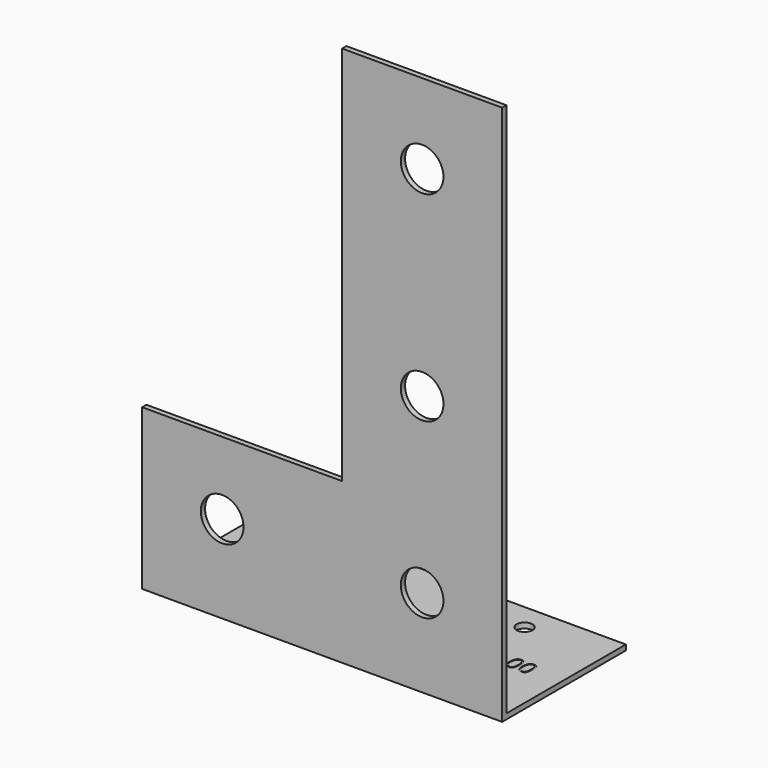
from build123d import *

# Parameters (mm, degrees)
F0_R         = 4
F0_W         = 67.5
F0_H         = 1
F1_DEPTH     = 1
F2_DEPTH     = 28
F3_R         = 1.5
F4_DEPTH     = 1
F5_TEXT_SIZE = 4.1666666667
F6_DEPTH     = 0.1


# Not quite as in the source:
# - Text() gives the source's letters only with a copy of the font that has no kerning and outlines rounded to 1/6400 em; it was checked with that copy


with BuildPart() as f1:
    # F0 (on Front) → F1 (new body)
    with BuildSketch(Plane.XZ):
        Polygon((0, 0), (-37.5, 0), (-37.5, -29), (30, -29), (30, 71.4), (0, 71.4), align=None)
        with Locations((-22.5, -13.6)):
            Circle(F0_R, mode=Mode.SUBTRACT)
        with Locations((15, -13.6)):
            Circle(F0_R, mode=Mode.SUBTRACT)
        with Locations((15, 18.9)):
            Circle(F0_R, mode=Mode.SUBTRACT)
        with Locations((15, 56.4)):
            Circle(F0_R, mode=Mode.SUBTRACT)
        with Locations((-3.75, -29.5)):
            Rectangle(F0_W, F0_H)
    extrude(amount=F1_DEPTH)

    # F0 (on Front) → F2 (join)
    with BuildSketch(Plane.XZ):
        with Locations((-3.75, -29.5)):
            Rectangle(F0_W, F0_H)
    extrude(amount=-F2_DEPTH)

    # F3 (on face) → F4 (cut, through all)
    with BuildSketch(Plane.XY.offset(-29)):
        with Locations((-22.5, 23)):
            Circle(F3_R)
        with Locations((15, 23)):
            Circle(F3_R)
    extrude(amount=-F4_DEPTH, mode=Mode.SUBTRACT)

    # F5 (on face) → F6 (cut)
    with BuildSketch(Plane.XY.offset(-29)):
        with Locations((-32.1365136172, 11.6149646826)):
            Text('Poti-Haltewinkel - 602-001-00', F5_TEXT_SIZE, font='Open Sans', text_align=(TextAlign.LEFT, TextAlign.BOTTOM))
    extrude(amount=-F6_DEPTH, mode=Mode.SUBTRACT)


solid = f1.part
